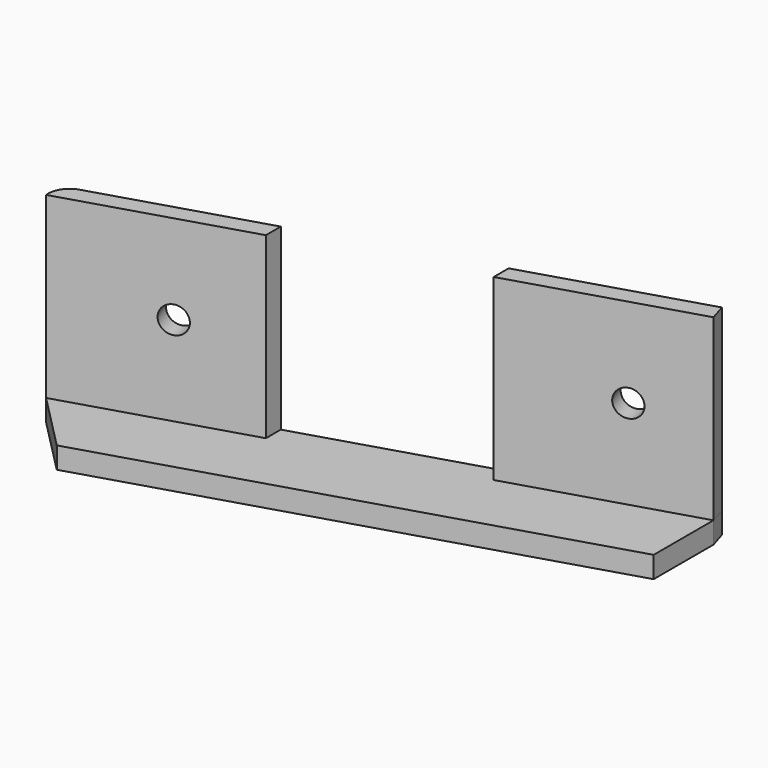
from build123d import *

# Parameters (mm, degrees)
F0_W         = 25
F0_H         = 33
F1_DEPTH     = 25
F3_DEPTH     = 10
F5_DEPTH     = 81.7
F7_DEPTH     = 10
F9_DEPTH     = 92
F10_W        = 13
F10_H        = 13
F11_DEPTH    = 40
F12_R        = 1.9
F13_DEPTH    = 7
F15_DEPTH    = 2.5
F16_W        = 78.4268817365
F16_H        = 25
F17_DEPTH    = 2.5
F19_DEPTH    = 336
F21_DEPTH    = 25
F23_W        = 90.9570492804
F23_H        = 10.3441323154
F24_DEPTH    = 48.1
F26_DEPTH    = 199
F27_W        = 183.3121031523
F27_H        = 83.9067064226
F28_DEPTH    = 179
F29_T1_DEPTH = 32.3950995948
F29_T3_DEPTH = 10.395099863
F31_DEPTH    = 25
F32_R        = 1.9
F33_DEPTH    = 25


# Not quite as in the source:
# - a fillet or chamfer that OpenCascade refuses, or shapes differently, is made with other operations: its cross-section is extruded or revolved along the edge and cut away or added


with BuildPart() as f1:
    # F0 (on Top) → F1 (new body)
    with BuildSketch(Plane.XY):
        with Locations((12.5, 16.5)):
            Rectangle(F0_W, F0_H)
        Polygon((-25, 25.3567329635), (0, 0), (0, 33), align=None)
        with Locations((37.5, 16.5)):
            Rectangle(F0_W, F0_H)
        Polygon((25, 40.6432670365), (0, 33), (25, 33), align=None)
        Polygon((0, 101.4598330308), (0, 33), (25, 40.6432670365), (25, 101.4598330308), (25, 137), (0, 137), align=None)
        Polygon((25, 40.6432670365), (25, 33), (50, 33), (50, 48.2865340729), align=None)
        Polygon((-25, 131.6860859582), (0, 101.4598330308), (0, 137), align=None)
        Polygon((25, 137), (25, 101.4598330308), (50, 131.6860859582), (50, 147.6278280835), (25, 142.3139140418), align=None)
        Polygon((25, 142.3139140418), (0, 137), (25, 137), align=None)
        Polygon((0, 177), (0, 137), (25, 142.3139140418), (25, 177), align=None)
    extrude(amount=F1_DEPTH)

    # F2 (on face) → F3 (join)
    with BuildSketch(Plane(origin=(0, 0, 0), x_dir=(1, 0, 0), z_dir=(0, 0, -1))):
        Polygon((50, -131.6860859582), (25, -101.4598330308), (0, -101.4598330308), (-25, -131.6860859582), (50, -147.6278280835), align=None)
    extrude(amount=F3_DEPTH)

    # F4 (on face) → F5 (cut, symmetric)
    with BuildSketch(Plane.YZ.offset(25)):
        Polygon((101.4598330308, -21.1370438337), (147.6278330308, -10), (101.4598330308, 0), align=None)
    extrude(amount=F5_DEPTH, both=True, mode=Mode.SUBTRACT)

    # F6 (on face) → F7 (join)
    with BuildSketch(Plane(origin=(0, 0, 0), x_dir=(1, 0, 0), z_dir=(0, 0, -1))):
        Polygon((50, -48.2865340729), (50, 0), (0, 0), (-25, -25.3567329635), align=None)
    extrude(amount=F7_DEPTH)

    # F8 (on face) → F9 (cut)
    with BuildSketch(Plane.YZ.offset(50)):
        Polygon((48.2865340729, -10), (0, 0), (0, -39.534393698), (48.2865340729, -39.534393698), align=None)
    extrude(amount=-F9_DEPTH, mode=Mode.SUBTRACT)

    # F10 (on face) → F11 (cut)
    with BuildSketch(Plane(origin=(0, 177, 0), x_dir=(-1, 0, 0), z_dir=(0, 1, 0))):
        with Locations((-12.5, 12.5)):
            Rectangle(F10_W, F10_H)
    extrude(amount=-F11_DEPTH, mode=Mode.SUBTRACT)

    # F12 (on face) → F13 (cut)
    with BuildSketch(Plane(origin=(-27.8614600507, 131.0778638485, 0), x_dir=(-0.9781476007, -0.2079116908, 0), z_dir=(-0.2079116908, 0.9781476007, 0))):
        with Locations((-18.6253867704, 12.5)):
            Circle(F12_R)
        with BuildLine():
            ThreePointArc((-72.2009313853, 12.5), (-70.3009313853, 10.6), (-68.4009313853, 12.5))
            ThreePointArc((-68.4009313853, 12.5), (-70.3009313853, 14.4), (-72.2009313853, 12.5))
        make_face()
    extrude(amount=-F13_DEPTH, mode=Mode.SUBTRACT)

    # F15 (add): a face of the model
    f15_faces = [f1.faces().sort_by_distance(p)[0] for p in [
        (12.5, 36.8216335182, -0.8588233683),
    ]]
    extrude(f15_faces, amount=F15_DEPTH)

    # F16 (on face) → F17 (join)
    with BuildSketch(Plane(origin=(-9.9576121691, 32.5698818371, 0), x_dir=(-0.956304756, -0.2923717047, 0), z_dir=(-0.2923717047, 0.956304756, 0))):
        with Locations((-22.7194132119, 12.5)):
            Rectangle(F16_W, F16_H)
    extrude(amount=-F17_DEPTH)

    # F18 (on face) → F19 (cut)
    with BuildSketch(Plane(origin=(-9.9576121691, 32.5698818371, 0), x_dir=(-0.956304756, -0.2923717047, 0), z_dir=(-0.2923717047, 0.956304756, 0))):
        Polygon((16.4940276563, -15.7148446888), (16.4940276563, -3), (-61.9328540802, -3), (-74.3611752987, -3), (-74.3611752987, -15.7148446888), align=None)
    extrude(amount=-F19_DEPTH, mode=Mode.SUBTRACT)

    # F20 (on face) → F21 (cut)
    with BuildSketch(Plane.XY.offset(25)):
        Polygon((50, 48.2865340729), (-25, 25.3567329635), (-20.5921567976, -5.8456440456), (63.7660473585, -9.7692795098), align=None)
    extrude(amount=-F21_DEPTH, mode=Mode.SUBTRACT)

    # F23 (on offset) → F24 (cut)
    with BuildSketch(Plane(origin=(-6.30296586, 20.6160723875, 0), x_dir=(-0.956304756, -0.2923717047, 0), z_dir=(-0.2923717047, 0.956304756, 0))):
        with Locations((-20.5792468041, -2.5766163599)):
            Rectangle(F23_W, F23_H)
    extrude(amount=-F24_DEPTH, mode=Mode.SUBTRACT)

    # F25 (on face) → F26 (cut)
    with BuildSketch(Plane(origin=(0, 177, 0), x_dir=(-1, 0, 0), z_dir=(0, 1, 0))):
        Polygon((0.3, 25), (0, 25), (-25, 25), (-25.3, 25), (-25.3, 0), (-25, 0), (0, 0), (0.3, 0), align=None)
    extrude(amount=-F26_DEPTH, mode=Mode.SUBTRACT)

    # F27 (on face) → F28 (cut)
    with BuildSketch(Plane(origin=(-9.9576121691, 32.5698818371, 0), x_dir=(-0.956304756, -0.2923717047, 0), z_dir=(-0.2923717047, 0.956304756, 0))):
        with Locations((-51.5790507197, 11.8016507477)):
            Rectangle(F27_W, F27_H)
    extrude(amount=F28_DEPTH, mode=Mode.SUBTRACT)

    # F29: fillet of radius 3 on 1 edges, made by hand

    # F29_s2 → F29_t1 (cut)
    with BuildSketch(Plane.XY.offset(1.341e-07)):
        with BuildLine():
            ThreePointArc((-25, 25.3567329635), (-24.5468104619, 27.3684218455), (-22.9021416452, 28.6123420192))
            Line((-22.9021416452, 28.6123420192), (-25.7309292618, 27.7474948534))
            Line((-25.7309292618, 27.7474948534), (-25, 25.3567329635))
        make_face()
    extrude(amount=F29_T1_DEPTH, mode=Mode.SUBTRACT)

    # F29_s4 → F29_t3 (cut)
    with BuildSketch(Plane.XY.offset(-10.3950997289)):
        with BuildLine():
            ThreePointArc((-25, 25.3567329635), (-24.5468104619, 27.3684218455), (-22.9021416452, 28.6123420192))
            Line((-22.9021416452, 28.6123420192), (-25.7309292618, 27.7474948534))
            Line((-25.7309292618, 27.7474948534), (-25, 25.3567329635))
        make_face()
    extrude(amount=F29_T3_DEPTH, mode=Mode.SUBTRACT)

    # F30 (on face) → F31 (cut)
    with BuildSketch(Plane(origin=(-9.2266829073, 30.1791199472, 0), x_dir=(0.956304756, 0.2923717047, 0), z_dir=(0.2923717047, -0.956304756, 0))):
        with BuildLine():
            ThreePointArc((-3.3940276563, 12.5), (-1.4940276563, 10.6), (0.4059723437, 12.5))
            ThreePointArc((0.4059723437, 12.5), (-1.4940276563, 14.4), (-3.3940276563, 12.5))
        make_face()
    extrude(amount=-F31_DEPTH, mode=Mode.SUBTRACT)

    # F32 (on face) → F33 (cut)
    with BuildSketch(Plane(origin=(-9.2266829073, 30.1791199472, 0), x_dir=(0.956304756, 0.2923717047, 0), z_dir=(0.2923717047, -0.956304756, 0))):
        with Locations((51.9328540802, 12.5)):
            Circle(F32_R)
    extrude(amount=-F33_DEPTH, mode=Mode.SUBTRACT)


solid = f1.part
